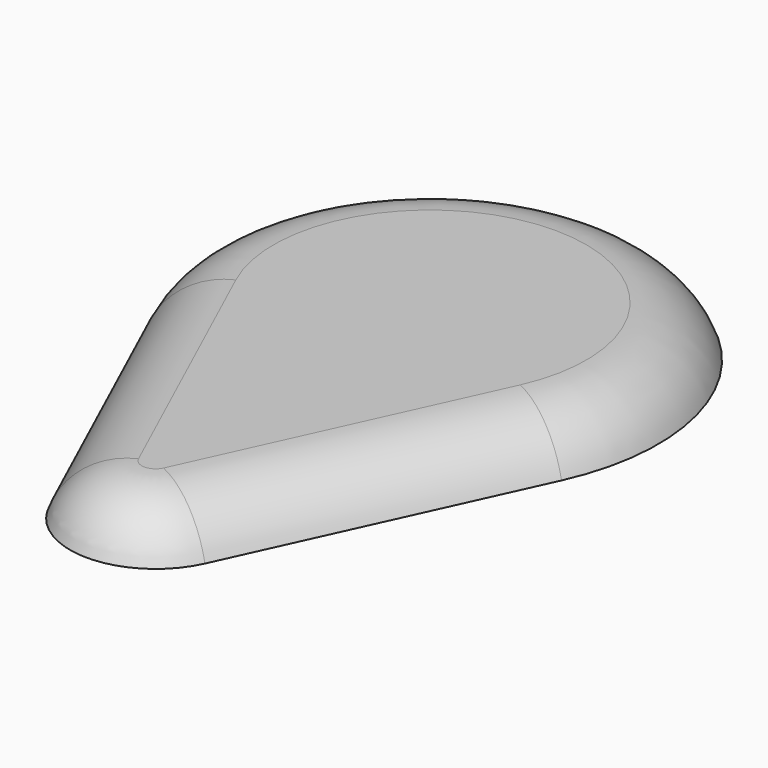
from build123d import *

# Parameters (mm, degrees)
F1_DEPTH    = 2
F2_T1_DEPTH = 12.292205585
F2_T3_DEPTH = 12.292205585
F2_T6_ANGLE = 229.1191340219
F2_T8_ANGLE = 130.8808659781


# Not quite as in the source:
# - a fillet or chamfer that OpenCascade refuses, or shapes differently, is made with other operations: its cross-section is extruded or revolved along the edge and cut away or added


with BuildPart() as f1:
    # F0 (on Top) → F1 (new body)
    with BuildSketch(Plane.XY):
        with BuildLine():
            Line((-8.1754417997, 2.5021668996), (-3.0663211364, -8.6779585108))
            ThreePointArc((-3.0663211364, -8.6779585108), (0, -10.648029893), (3.0663211364, -8.6779585108))
            Line((3.0663211364, -8.6779585108), (8.1754417997, 2.5021668996))
            ThreePointArc((8.1754417997, 2.5021668996), (0, 15.2268479526), (-8.1754417997, 2.5021668996))
        make_face()
    extrude(amount=F1_DEPTH)

    # F2: fillet of radius 3 on 4 edges, made by hand

    # F2_s2 → F2_t1 (cut)
    with BuildSketch(Plane(origin=(-2.7508562412, -6.0196107686, 0), x_dir=(0, 0, 1), z_dir=(0.4156390509, 0.9095296473, 0))):
        with BuildLine():
            ThreePointArc((0, 6.3958084213), (1.4494897428, 5.2994321041), (2, 3.5673812965))
            Line((2, 3.5673812965), (2, 6.3958084213))
            Line((2, 6.3958084213), (0, 6.3958084213))
        make_face()
    extrude(amount=F2_T1_DEPTH, mode=Mode.SUBTRACT)

    # F2_s4 → F2_t3 (cut)
    with BuildSketch(Plane(origin=(-2.358264422, 5.1605146418, 0), x_dir=(0, 0, 1), z_dir=(0.4156390509, -0.9095296473, 0))):
        with BuildLine():
            ThreePointArc((0, 6.3958084213), (1.4494897428, 5.2994321041), (2, 3.5673812965))
            Line((2, 3.5673812965), (2, 6.3958084213))
            Line((2, 6.3958084213), (0, 6.3958084213))
        make_face()
    extrude(amount=F2_T3_DEPTH, mode=Mode.SUBTRACT)

    # F2_s5 → F2_t6 (revolve, cut)
    with BuildSketch(Plane(origin=(2.358264422, 5.1605146418, 0), x_dir=(0, 0, 1), z_dir=(-0.4156390509, -0.9095296473, 0))):
        with BuildLine():
            ThreePointArc((0, -6.3958084213), (1.4494897428, -5.2994321041), (2, -3.5673812965))
            Line((2, -3.5673812965), (2, -6.3958084213))
            Line((2, -6.3958084213), (0, -6.3958084213))
        make_face()
    revolve(axis=Axis((0, 6.2382000027, 2), (0, 0, 1)), revolution_arc=F2_T6_ANGLE, mode=Mode.SUBTRACT)

    # F2_s7 → F2_t8 (revolve, cut)
    with BuildSketch(Plane(origin=(2.7508562412, -6.0196107686, 0), x_dir=(0, 0, 1), z_dir=(-0.4156390509, 0.9095296473, 0))):
        with BuildLine():
            ThreePointArc((0, -6.3958084213), (1.4494897428, -5.2994321041), (2, -3.5673812965))
            Line((2, -3.5673812965), (2, -6.3958084213))
            Line((2, -6.3958084213), (0, -6.3958084213))
        make_face()
    revolve(axis=Axis((0, -7.2767036856, 2), (0, 0, 1)), revolution_arc=F2_T8_ANGLE, mode=Mode.SUBTRACT)


solid = f1.part
